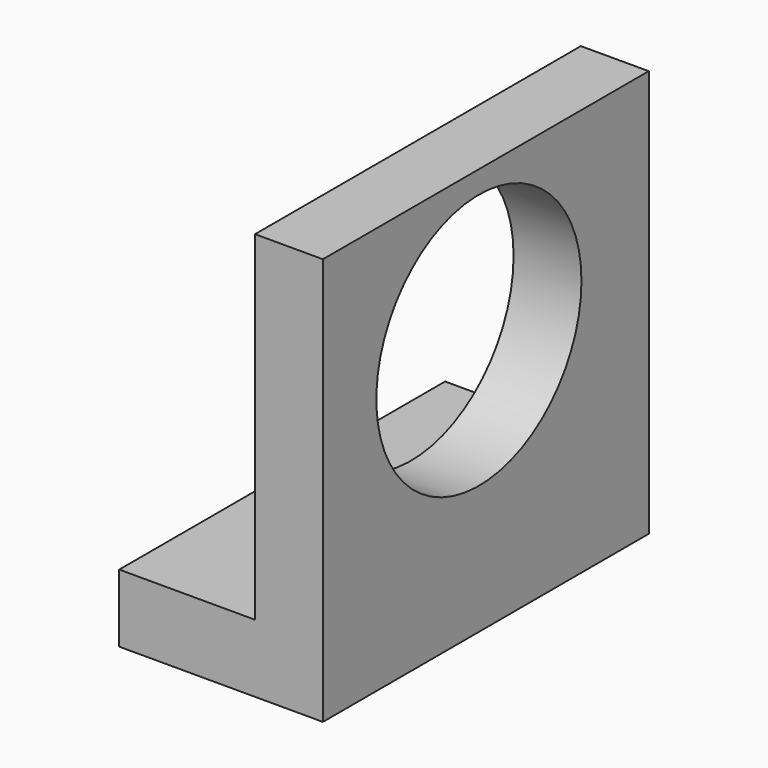
from build123d import *

# Parameters (mm, degrees)
F1_DEPTH = 152.4
F2_R     = 47.9646820368
F3_DEPTH = 152.4


# Not quite as in the source:
# - a feature names something its author has since deleted; it is built from what else it names


with BuildPart() as f1:
    # F0 (on Front) → F1 (new body)
    with BuildSketch(Plane.XZ):
        Polygon((-76.2, 0), (0, 0), (0, 152.4), (-25.4, 152.4), (-25.4, 25.4), (-76.2, 25.4), align=None)
    extrude(amount=-F1_DEPTH)

    # F2 (on Right) → F3 (cut)
    with BuildSketch(Plane.YZ):
        with Locations((72.9622766376, 96.0644483566)):
            Circle(F2_R)
    extrude(amount=-F3_DEPTH, mode=Mode.SUBTRACT)


solid = f1.part
